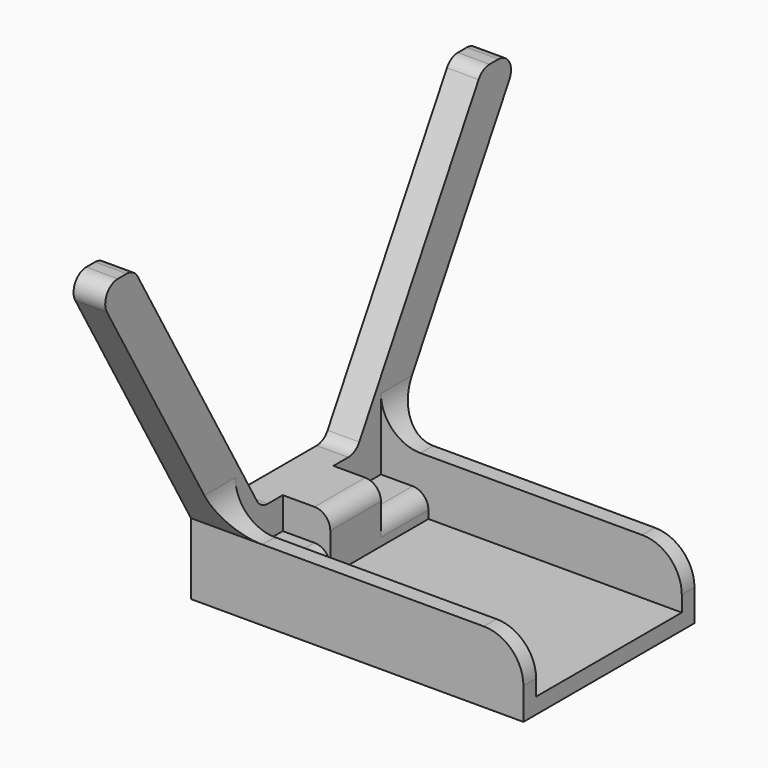
from build123d import *

# Parameters (mm, degrees)
F0_W      = 42
F0_H      = 27
F1_DEPTH  = 9
F2_W      = 32
F2_H      = 23
F3_DEPTH  = 7
F6_W      = 6
F6_H      = 7.5
F7_DEPTH  = 4
F5_W      = 6
F5_H      = 7.5
F10_DEPTH = 4
F12_DEPTH = 5
F14_R     = 2
F15_R     = 5


with BuildPart() as f1:
    # F0 (on Top) → F1 (new body)
    with BuildSketch(Plane.XY):
        Rectangle(F0_W, F0_H)
    extrude(amount=-F1_DEPTH)


with BuildPart() as f3:
    # F2 (on Top) → F3 (new body)
    with BuildSketch(Plane.XY):
        with Locations((5, 0)):
            Rectangle(F2_W, F2_H)
    extrude(amount=-F3_DEPTH)


with BuildPart() as f1_1:
    add(f1.part)

    # F4: cut F3
    add(f3.part, mode=Mode.SUBTRACT)


with BuildPart() as f7:
    # F6 (on Top) → F7 (new body)
    with BuildSketch(Plane.XY):
        with Locations((-14, -7.75)):
            Rectangle(F6_W, F6_H)
    extrude(amount=-F7_DEPTH)


with BuildPart() as f7b:
    # F5 (on Top) → F7, piece 2 (new body)
    with BuildSketch(Plane.XY):
        with Locations((-14, 7.75)):
            Rectangle(F5_W, F5_H)
    extrude(amount=-F7_DEPTH)


with BuildPart() as f1_2:
    add(f1_1.part)

    # F8: cut F7b, F7
    add(f7b.part, mode=Mode.SUBTRACT)
    add(f7.part, mode=Mode.SUBTRACT)

    # F9 (on face) → F10 (join)
    with BuildSketch(Plane(origin=(-21, 0, 0), x_dir=(0, -1, 0), z_dir=(-1, 0, 0))):
        Polygon((-13.5, 0), (13.5, 0), (33.5, 34.6410161514), (-33.5, 34.6410161514), align=None)
    extrude(amount=-F10_DEPTH)


with BuildPart() as f12:
    # F11 (on face) → F12 (new body)
    with BuildSketch(Plane(origin=(-21, 0, 0), x_dir=(0, -1, 0), z_dir=(-1, 0, 0))):
        Polygon((-7.5, 0), (7.5, 0), (27.5, 34.6410161514), (-27.5, 34.6410161514), align=None)
    extrude(amount=-F12_DEPTH)


with BuildPart() as f1_3:
    add(f1_2.part)

    # F13: cut F12
    add(f12.part, mode=Mode.SUBTRACT)

    # F14
    f14_edges = [f1_3.edges().sort_by_distance(p)[0] for p in [
        (-19, 33.5, 34.641016),
        (-19, 27.5, 34.641016),
        (-19, -27.5, 34.641016),
        (-19, -33.5, 34.641016),
        (-19, -7.5, 0),
        (-19, 7.5, 0),
        (-11, 0, 0),
        (-11, 7.75, -4),
        (-11, -7.75, -4),
    ]]
    fillet(f14_edges, radius=F14_R)

    # F15
    f15_edges = [f1_3.edges().sort_by_distance(p)[0] for p in [
        (-17, -12.5, 0),
        (-17, 12.5, 0),
        (21, 12.5, 0),
        (21, -12.5, 0),
    ]]
    fillet(f15_edges, radius=F15_R)


solid = f1_3.part
